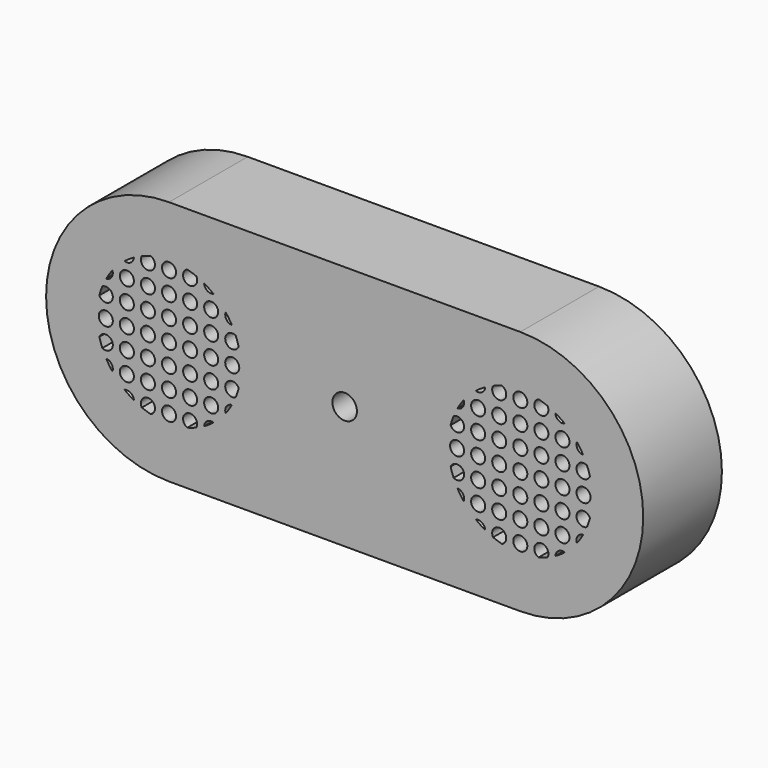
from build123d import *

# Parameters (mm, degrees)
F0_R     = 20.5
F0_R_2   = 3.5
F1_DEPTH = 3
F2_R     = 3.5
F2_R_2   = 2
F3_DEPTH = 25


# Not quite as in the source:
# - after a boolean that leaves OpenCascade's solid faulty, fix() repairs it


with BuildPart() as f1:
    # F0 (on Front) → F1 (new body)
    with BuildSketch(Plane.XZ):
        with BuildLine():
            ThreePointArc((-50, 35), (-85, 0), (-50, -35))
            Line((-50, -35), (50, -35))
            ThreePointArc((50, -35), (85, 0), (50, 35))
            Line((50, 35), (-50, 35))
        make_face()
        with Locations((-50, 0)):
            Circle(F0_R, mode=Mode.SUBTRACT)
        Circle(F0_R_2, mode=Mode.SUBTRACT)
        with Locations((50, 0)):
            Circle(F0_R, mode=Mode.SUBTRACT)
    extrude(amount=F1_DEPTH)

    # F2 (on face) → F3 (join)
    with BuildSketch(Plane.XZ.offset(3)):
        with BuildLine():
            ThreePointArc((50, -35), (85, 0), (50, 35))
            Line((50, 35), (-50, 35))
            ThreePointArc((-50, 35), (-85, 0), (-50, -35))
            Line((-50, -35), (50, -35))
        make_face()
        with BuildLine():
            ThreePointArc((-32.1060421417, 10.0028132125), (-31.5275850928, 8.889313106), (-31.0183361956, 7.7425085868))
            ThreePointArc((-31.0183361956, 7.7425085868), (-30.55199239, 6.4826692033), (-30.1691638044, 5.1949914132))
            ThreePointArc((-30.1691638044, 5.1949914132), (-29.6679791707, 2.618955707), (-29.5, 0))
            ThreePointArc((-29.5, 0), (-29.6679791707, -2.618955707), (-30.1691638044, -5.1949914132))
            ThreePointArc((-30.1691638044, -5.1949914132), (-30.55199239, -6.4826692033), (-31.0183361956, -7.7425085868))
            ThreePointArc((-31.0183361956, -7.7425085868), (-31.5275850928, -8.889313106), (-32.1060421417, -10.0028132125))
            ThreePointArc((-32.1060421417, -10.0028132125), (-32.9429689661, -11.3713540226), (-33.8843424737, -12.6702637106))
            ThreePointArc((-33.8843424737, -12.6702637106), (-35.5043109857, -14.4956890143), (-37.3297362894, -16.1156575263))
            ThreePointArc((-37.3297362894, -16.1156575263), (-38.6286459774, -17.0570310339), (-39.9971867875, -17.8939578583))
            ThreePointArc((-39.9971867875, -17.8939578583), (-41.110686894, -18.4724149072), (-42.2574914132, -18.9816638044))
            ThreePointArc((-42.2574914132, -18.9816638044), (-43.5173307967, -19.44800761), (-44.8050085868, -19.8308361956))
            ThreePointArc((-44.8050085868, -19.8308361956), (-50, -20.5), (-55.1949914132, -19.8308361956))
            ThreePointArc((-55.1949914132, -19.8308361956), (-56.4826692033, -19.44800761), (-57.7425085868, -18.9816638044))
            ThreePointArc((-57.7425085868, -18.9816638044), (-58.889313106, -18.4724149072), (-60.0028132125, -17.8939578583))
            ThreePointArc((-60.0028132125, -17.8939578583), (-61.3713540226, -17.0570310339), (-62.6702637106, -16.1156575263))
            ThreePointArc((-62.6702637106, -16.1156575263), (-64.4956890143, -14.4956890143), (-66.1156575263, -12.6702637106))
            ThreePointArc((-66.1156575263, -12.6702637106), (-67.0570310339, -11.3713540226), (-67.8939578583, -10.0028132125))
            ThreePointArc((-67.8939578583, -10.0028132125), (-68.4724149072, -8.889313106), (-68.9816638044, -7.7425085868))
            ThreePointArc((-68.9816638044, -7.7425085868), (-69.44800761, -6.4826692033), (-69.8308361956, -5.1949914132))
            ThreePointArc((-69.8308361956, -5.1949914132), (-70.5, 0), (-69.8308361956, 5.1949914132))
            ThreePointArc((-69.8308361956, 5.1949914132), (-69.44800761, 6.4826692033), (-68.9816638044, 7.7425085868))
            ThreePointArc((-68.9816638044, 7.7425085868), (-68.4724149072, 8.889313106), (-67.8939578583, 10.0028132125))
            ThreePointArc((-67.8939578583, 10.0028132125), (-67.0570310339, 11.3713540226), (-66.1156575263, 12.6702637106))
            ThreePointArc((-66.1156575263, 12.6702637106), (-64.4956890143, 14.4956890143), (-62.6702637106, 16.1156575263))
            ThreePointArc((-62.6702637106, 16.1156575263), (-61.3713540226, 17.0570310339), (-60.0028132125, 17.8939578583))
            ThreePointArc((-60.0028132125, 17.8939578583), (-58.889313106, 18.4724149072), (-57.7425085868, 18.9816638044))
            ThreePointArc((-57.7425085868, 18.9816638044), (-56.4826692033, 19.44800761), (-55.1949914132, 19.8308361956))
            ThreePointArc((-55.1949914132, 19.8308361956), (-50, 20.5), (-44.8050085868, 19.8308361956))
            ThreePointArc((-44.8050085868, 19.8308361956), (-43.5173307967, 19.44800761), (-42.2574914132, 18.9816638044))
            ThreePointArc((-42.2574914132, 18.9816638044), (-41.110686894, 18.4724149072), (-39.9971867875, 17.8939578583))
            ThreePointArc((-39.9971867875, 17.8939578583), (-38.6286459774, 17.0570310339), (-37.3297362894, 16.1156575263))
            ThreePointArc((-37.3297362894, 16.1156575263), (-35.5043109857, 14.4956890143), (-33.8843424737, 12.6702637106))
            ThreePointArc((-33.8843424737, 12.6702637106), (-32.9429689661, 11.3713540226), (-32.1060421417, 10.0028132125))
        make_face(mode=Mode.SUBTRACT)
        Circle(F2_R, mode=Mode.SUBTRACT)
        with BuildLine():
            ThreePointArc((57.7425085868, 18.9816638044), (58.889313106, 18.4724149072), (60.0028132125, 17.8939578583))
            ThreePointArc((60.0028132125, 17.8939578583), (61.3713540226, 17.0570310339), (62.6702637106, 16.1156575263))
            ThreePointArc((62.6702637106, 16.1156575263), (64.4956890143, 14.4956890143), (66.1156575263, 12.6702637106))
            ThreePointArc((66.1156575263, 12.6702637106), (67.0570310339, 11.3713540226), (67.8939578583, 10.0028132125))
            ThreePointArc((67.8939578583, 10.0028132125), (68.4724149072, 8.889313106), (68.9816638044, 7.7425085868))
            ThreePointArc((68.9816638044, 7.7425085868), (69.44800761, 6.4826692033), (69.8308361956, 5.1949914132))
            ThreePointArc((69.8308361956, 5.1949914132), (70.3320208293, 2.618955707), (70.5, 0))
            ThreePointArc((70.5, 0), (70.3320208293, -2.618955707), (69.8308361956, -5.1949914132))
            ThreePointArc((69.8308361956, -5.1949914132), (69.44800761, -6.4826692033), (68.9816638044, -7.7425085868))
            ThreePointArc((68.9816638044, -7.7425085868), (68.4724149072, -8.889313106), (67.8939578583, -10.0028132125))
            ThreePointArc((67.8939578583, -10.0028132125), (67.0570310339, -11.3713540226), (66.1156575263, -12.6702637106))
            ThreePointArc((66.1156575263, -12.6702637106), (64.4956890143, -14.4956890143), (62.6702637106, -16.1156575263))
            ThreePointArc((62.6702637106, -16.1156575263), (61.3713540226, -17.0570310339), (60.0028132125, -17.8939578583))
            ThreePointArc((60.0028132125, -17.8939578583), (58.889313106, -18.4724149072), (57.7425085868, -18.9816638044))
            ThreePointArc((57.7425085868, -18.9816638044), (56.4826692033, -19.44800761), (55.1949914132, -19.8308361956))
            ThreePointArc((55.1949914132, -19.8308361956), (50, -20.5), (44.8050085868, -19.8308361956))
            ThreePointArc((44.8050085868, -19.8308361956), (43.5173307967, -19.44800761), (42.2574914132, -18.9816638044))
            ThreePointArc((42.2574914132, -18.9816638044), (41.110686894, -18.4724149072), (39.9971867875, -17.8939578583))
            ThreePointArc((39.9971867875, -17.8939578583), (38.6286459774, -17.0570310339), (37.3297362894, -16.1156575263))
            ThreePointArc((37.3297362894, -16.1156575263), (35.5043109857, -14.4956890143), (33.8843424737, -12.6702637106))
            ThreePointArc((33.8843424737, -12.6702637106), (32.9429689661, -11.3713540226), (32.1060421417, -10.0028132125))
            ThreePointArc((32.1060421417, -10.0028132125), (31.5275850928, -8.889313106), (31.0183361956, -7.7425085868))
            ThreePointArc((31.0183361956, -7.7425085868), (30.55199239, -6.4826692033), (30.1691638044, -5.1949914132))
            ThreePointArc((30.1691638044, -5.1949914132), (29.5, 0), (30.1691638044, 5.1949914132))
            ThreePointArc((30.1691638044, 5.1949914132), (30.55199239, 6.4826692033), (31.0183361956, 7.7425085868))
            ThreePointArc((31.0183361956, 7.7425085868), (31.5275850928, 8.889313106), (32.1060421417, 10.0028132125))
            ThreePointArc((32.1060421417, 10.0028132125), (32.9429689661, 11.3713540226), (33.8843424737, 12.6702637106))
            ThreePointArc((33.8843424737, 12.6702637106), (35.5043109857, 14.4956890143), (37.3297362894, 16.1156575263))
            ThreePointArc((37.3297362894, 16.1156575263), (38.6286459774, 17.0570310339), (39.9971867875, 17.8939578583))
            ThreePointArc((39.9971867875, 17.8939578583), (41.110686894, 18.4724149072), (42.2574914132, 18.9816638044))
            ThreePointArc((42.2574914132, 18.9816638044), (43.5173307967, 19.44800761), (44.8050085868, 19.8308361956))
            ThreePointArc((44.8050085868, 19.8308361956), (50, 20.5), (55.1949914132, 19.8308361956))
            ThreePointArc((55.1949914132, 19.8308361956), (56.4826692033, 19.44800761), (57.7425085868, 18.9816638044))
        make_face(mode=Mode.SUBTRACT)
        with BuildLine():
            ThreePointArc((-30.1691638044, 5.1949914132), (-33.8973665961, 5.367544468), (-31.0183361956, 7.7425085868))
            ThreePointArc((-31.0183361956, 7.7425085868), (-31.5275850928, 8.889313106), (-32.1060421417, 10.0028132125))
            ThreePointArc((-32.1060421417, 10.0028132125), (-33.6641005887, 10.8905996075), (-33.8843424737, 12.6702637106))
            ThreePointArc((-33.8843424737, 12.6702637106), (-35.5043109857, 14.4956890143), (-37.3297362894, 16.1156575263))
            ThreePointArc((-37.3297362894, 16.1156575263), (-39.1094003925, 16.3358994113), (-39.9971867875, 17.8939578583))
            ThreePointArc((-39.9971867875, 17.8939578583), (-41.110686894, 18.4724149072), (-42.2574914132, 18.9816638044))
            ThreePointArc((-42.2574914132, 18.9816638044), (-44.632455532, 16.1026334039), (-44.8050085868, 19.8308361956))
            ThreePointArc((-44.8050085868, 19.8308361956), (-50, 20.5), (-55.1949914132, 19.8308361956))
            ThreePointArc((-55.1949914132, 19.8308361956), (-55.367544468, 16.1026334039), (-57.7425085868, 18.9816638044))
            ThreePointArc((-57.7425085868, 18.9816638044), (-58.889313106, 18.4724149072), (-60.0028132125, 17.8939578583))
            ThreePointArc((-60.0028132125, 17.8939578583), (-60.8905996075, 16.3358994113), (-62.6702637106, 16.1156575263))
            ThreePointArc((-62.6702637106, 16.1156575263), (-64.4956890143, 14.4956890143), (-66.1156575263, 12.6702637106))
            ThreePointArc((-66.1156575263, 12.6702637106), (-66.3358994113, 10.8905996075), (-67.8939578583, 10.0028132125))
            ThreePointArc((-67.8939578583, 10.0028132125), (-68.4724149072, 8.889313106), (-68.9816638044, 7.7425085868))
            ThreePointArc((-68.9816638044, 7.7425085868), (-66.1026334039, 5.367544468), (-69.8308361956, 5.1949914132))
            ThreePointArc((-69.8308361956, 5.1949914132), (-70.5, 0), (-69.8308361956, -5.1949914132))
            ThreePointArc((-69.8308361956, -5.1949914132), (-66.1026334039, -5.367544468), (-68.9816638044, -7.7425085868))
            ThreePointArc((-68.9816638044, -7.7425085868), (-68.4724149072, -8.889313106), (-67.8939578583, -10.0028132125))
            ThreePointArc((-67.8939578583, -10.0028132125), (-66.3358994113, -10.8905996075), (-66.1156575263, -12.6702637106))
            ThreePointArc((-66.1156575263, -12.6702637106), (-64.4956890143, -14.4956890143), (-62.6702637106, -16.1156575263))
            ThreePointArc((-62.6702637106, -16.1156575263), (-60.8905996075, -16.3358994113), (-60.0028132125, -17.8939578583))
            ThreePointArc((-60.0028132125, -17.8939578583), (-58.889313106, -18.4724149072), (-57.7425085868, -18.9816638044))
            ThreePointArc((-57.7425085868, -18.9816638044), (-55.367544468, -16.1026334039), (-55.1949914132, -19.8308361956))
            ThreePointArc((-55.1949914132, -19.8308361956), (-50, -20.5), (-44.8050085868, -19.8308361956))
            ThreePointArc((-44.8050085868, -19.8308361956), (-44.632455532, -16.1026334039), (-42.2574914132, -18.9816638044))
            ThreePointArc((-42.2574914132, -18.9816638044), (-41.110686894, -18.4724149072), (-39.9971867875, -17.8939578583))
            ThreePointArc((-39.9971867875, -17.8939578583), (-39.1094003925, -16.3358994113), (-37.3297362894, -16.1156575263))
            ThreePointArc((-37.3297362894, -16.1156575263), (-35.5043109857, -14.4956890143), (-33.8843424737, -12.6702637106))
            ThreePointArc((-33.8843424737, -12.6702637106), (-33.6641005887, -10.8905996075), (-32.1060421417, -10.0028132125))
            ThreePointArc((-32.1060421417, -10.0028132125), (-31.5275850928, -8.889313106), (-31.0183361956, -7.7425085868))
            ThreePointArc((-31.0183361956, -7.7425085868), (-33.8973665961, -5.367544468), (-30.1691638044, -5.1949914132))
            ThreePointArc((-30.1691638044, -5.1949914132), (-29.6679791707, -2.618955707), (-29.5, 0))
            ThreePointArc((-29.5, 0), (-29.6679791707, 2.618955707), (-30.1691638044, 5.1949914132))
        make_face()
        with Locations((-50, -18)):
            Circle(F2_R_2, mode=Mode.SUBTRACT)
        with Locations((-62, -12)):
            Circle(F2_R_2, mode=Mode.SUBTRACT)
        with Locations((-56, -12)):
            Circle(F2_R_2, mode=Mode.SUBTRACT)
        with Locations((-50, -12)):
            Circle(F2_R_2, mode=Mode.SUBTRACT)
        with Locations((-44, -12)):
            Circle(F2_R_2, mode=Mode.SUBTRACT)
        with Locations((-62, -6)):
            Circle(F2_R_2, mode=Mode.SUBTRACT)
        with Locations((-56, -6)):
            Circle(F2_R_2, mode=Mode.SUBTRACT)
        with Locations((-50, -6)):
            Circle(F2_R_2, mode=Mode.SUBTRACT)
        with Locations((-44, -6)):
            Circle(F2_R_2, mode=Mode.SUBTRACT)
        with Locations((-38, -12)):
            Circle(F2_R_2, mode=Mode.SUBTRACT)
        with Locations((-38, -6)):
            Circle(F2_R_2, mode=Mode.SUBTRACT)
        with Locations((-68, 0)):
            Circle(F2_R_2, mode=Mode.SUBTRACT)
        with Locations((-62, 0)):
            Circle(F2_R_2, mode=Mode.SUBTRACT)
        with Locations((-56, 0)):
            Circle(F2_R_2, mode=Mode.SUBTRACT)
        with Locations((-50, 0)):
            Circle(F2_R_2, mode=Mode.SUBTRACT)
        with Locations((-44, 0)):
            Circle(F2_R_2, mode=Mode.SUBTRACT)
        with Locations((-62, 6)):
            Circle(F2_R_2, mode=Mode.SUBTRACT)
        with Locations((-56, 6)):
            Circle(F2_R_2, mode=Mode.SUBTRACT)
        with Locations((-50, 6)):
            Circle(F2_R_2, mode=Mode.SUBTRACT)
        with Locations((-44, 6)):
            Circle(F2_R_2, mode=Mode.SUBTRACT)
        with Locations((-62, 12)):
            Circle(F2_R_2, mode=Mode.SUBTRACT)
        with Locations((-56, 12)):
            Circle(F2_R_2, mode=Mode.SUBTRACT)
        with Locations((-50, 12)):
            Circle(F2_R_2, mode=Mode.SUBTRACT)
        with Locations((-44, 12)):
            Circle(F2_R_2, mode=Mode.SUBTRACT)
        with Locations((-38, 0)):
            Circle(F2_R_2, mode=Mode.SUBTRACT)
        with Locations((-32, 0)):
            Circle(F2_R_2, mode=Mode.SUBTRACT)
        with Locations((-38, 6)):
            Circle(F2_R_2, mode=Mode.SUBTRACT)
        with Locations((-38, 12)):
            Circle(F2_R_2, mode=Mode.SUBTRACT)
        with Locations((-50, 18)):
            Circle(F2_R_2, mode=Mode.SUBTRACT)
        with BuildLine():
            ThreePointArc((62.6702637106, 16.1156575263), (60.8905996075, 16.3358994113), (60.0028132125, 17.8939578583))
            ThreePointArc((60.0028132125, 17.8939578583), (58.889313106, 18.4724149072), (57.7425085868, 18.9816638044))
            ThreePointArc((57.7425085868, 18.9816638044), (55.367544468, 16.1026334039), (55.1949914132, 19.8308361956))
            ThreePointArc((55.1949914132, 19.8308361956), (50, 20.5), (44.8050085868, 19.8308361956))
            ThreePointArc((44.8050085868, 19.8308361956), (44.632455532, 16.1026334039), (42.2574914132, 18.9816638044))
            ThreePointArc((42.2574914132, 18.9816638044), (41.110686894, 18.4724149072), (39.9971867875, 17.8939578583))
            ThreePointArc((39.9971867875, 17.8939578583), (39.1094003925, 16.3358994113), (37.3297362894, 16.1156575263))
            ThreePointArc((37.3297362894, 16.1156575263), (35.5043109857, 14.4956890143), (33.8843424737, 12.6702637106))
            ThreePointArc((33.8843424737, 12.6702637106), (33.6641005887, 10.8905996075), (32.1060421417, 10.0028132125))
            ThreePointArc((32.1060421417, 10.0028132125), (31.5275850928, 8.889313106), (31.0183361956, 7.7425085868))
            ThreePointArc((31.0183361956, 7.7425085868), (33.8973665961, 5.367544468), (30.1691638044, 5.1949914132))
            ThreePointArc((30.1691638044, 5.1949914132), (29.5, 0), (30.1691638044, -5.1949914132))
            ThreePointArc((30.1691638044, -5.1949914132), (33.8973665961, -5.367544468), (31.0183361956, -7.7425085868))
            ThreePointArc((31.0183361956, -7.7425085868), (31.5275850928, -8.889313106), (32.1060421417, -10.0028132125))
            ThreePointArc((32.1060421417, -10.0028132125), (33.6641005887, -10.8905996075), (33.8843424737, -12.6702637106))
            ThreePointArc((33.8843424737, -12.6702637106), (35.5043109857, -14.4956890143), (37.3297362894, -16.1156575263))
            ThreePointArc((37.3297362894, -16.1156575263), (39.1094003925, -16.3358994113), (39.9971867875, -17.8939578583))
            ThreePointArc((39.9971867875, -17.8939578583), (41.110686894, -18.4724149072), (42.2574914132, -18.9816638044))
            ThreePointArc((42.2574914132, -18.9816638044), (44.632455532, -16.1026334039), (44.8050085868, -19.8308361956))
            ThreePointArc((44.8050085868, -19.8308361956), (50, -20.5), (55.1949914132, -19.8308361956))
            ThreePointArc((55.1949914132, -19.8308361956), (55.367544468, -16.1026334039), (57.7425085868, -18.9816638044))
            ThreePointArc((57.7425085868, -18.9816638044), (58.889313106, -18.4724149072), (60.0028132125, -17.8939578583))
            ThreePointArc((60.0028132125, -17.8939578583), (60.8905996075, -16.3358994113), (62.6702637106, -16.1156575263))
            ThreePointArc((62.6702637106, -16.1156575263), (64.4956890143, -14.4956890143), (66.1156575263, -12.6702637106))
            ThreePointArc((66.1156575263, -12.6702637106), (66.3358994113, -10.8905996075), (67.8939578583, -10.0028132125))
            ThreePointArc((67.8939578583, -10.0028132125), (68.4724149072, -8.889313106), (68.9816638044, -7.7425085868))
            ThreePointArc((68.9816638044, -7.7425085868), (66.1026334039, -5.367544468), (69.8308361956, -5.1949914132))
            ThreePointArc((69.8308361956, -5.1949914132), (70.3320208293, -2.618955707), (70.5, 0))
            ThreePointArc((70.5, 0), (70.3320208293, 2.618955707), (69.8308361956, 5.1949914132))
            ThreePointArc((69.8308361956, 5.1949914132), (66.1026334039, 5.367544468), (68.9816638044, 7.7425085868))
            ThreePointArc((68.9816638044, 7.7425085868), (68.4724149072, 8.889313106), (67.8939578583, 10.0028132125))
            ThreePointArc((67.8939578583, 10.0028132125), (66.3358994113, 10.8905996075), (66.1156575263, 12.6702637106))
            ThreePointArc((66.1156575263, 12.6702637106), (64.4956890143, 14.4956890143), (62.6702637106, 16.1156575263))
        make_face()
        with Locations((50, -18)):
            Circle(F2_R_2, mode=Mode.SUBTRACT)
        with Locations((38, -12)):
            Circle(F2_R_2, mode=Mode.SUBTRACT)
        with Locations((38, -6)):
            Circle(F2_R_2, mode=Mode.SUBTRACT)
        with Locations((44, -12)):
            Circle(F2_R_2, mode=Mode.SUBTRACT)
        with Locations((50, -12)):
            Circle(F2_R_2, mode=Mode.SUBTRACT)
        with Locations((56, -12)):
            Circle(F2_R_2, mode=Mode.SUBTRACT)
        with Locations((62, -12)):
            Circle(F2_R_2, mode=Mode.SUBTRACT)
        with Locations((44, -6)):
            Circle(F2_R_2, mode=Mode.SUBTRACT)
        with Locations((50, -6)):
            Circle(F2_R_2, mode=Mode.SUBTRACT)
        with Locations((56, -6)):
            Circle(F2_R_2, mode=Mode.SUBTRACT)
        with Locations((62, -6)):
            Circle(F2_R_2, mode=Mode.SUBTRACT)
        with Locations((32, 0)):
            Circle(F2_R_2, mode=Mode.SUBTRACT)
        with Locations((38, 0)):
            Circle(F2_R_2, mode=Mode.SUBTRACT)
        with Locations((38, 6)):
            Circle(F2_R_2, mode=Mode.SUBTRACT)
        with Locations((38, 12)):
            Circle(F2_R_2, mode=Mode.SUBTRACT)
        with Locations((44, 0)):
            Circle(F2_R_2, mode=Mode.SUBTRACT)
        with Locations((50, 0)):
            Circle(F2_R_2, mode=Mode.SUBTRACT)
        with Locations((56, 0)):
            Circle(F2_R_2, mode=Mode.SUBTRACT)
        with Locations((62, 0)):
            Circle(F2_R_2, mode=Mode.SUBTRACT)
        with Locations((44, 6)):
            Circle(F2_R_2, mode=Mode.SUBTRACT)
        with Locations((50, 6)):
            Circle(F2_R_2, mode=Mode.SUBTRACT)
        with Locations((56, 6)):
            Circle(F2_R_2, mode=Mode.SUBTRACT)
        with Locations((62, 6)):
            Circle(F2_R_2, mode=Mode.SUBTRACT)
        with Locations((68, 0)):
            Circle(F2_R_2, mode=Mode.SUBTRACT)
        with Locations((44, 12)):
            Circle(F2_R_2, mode=Mode.SUBTRACT)
        with Locations((50, 12)):
            Circle(F2_R_2, mode=Mode.SUBTRACT)
        with Locations((56, 12)):
            Circle(F2_R_2, mode=Mode.SUBTRACT)
        with Locations((62, 12)):
            Circle(F2_R_2, mode=Mode.SUBTRACT)
        with Locations((50, 18)):
            Circle(F2_R_2, mode=Mode.SUBTRACT)
    extrude(amount=F3_DEPTH)

    add(f1.part.fix(), mode=Mode.REPLACE)


solid = f1.part
